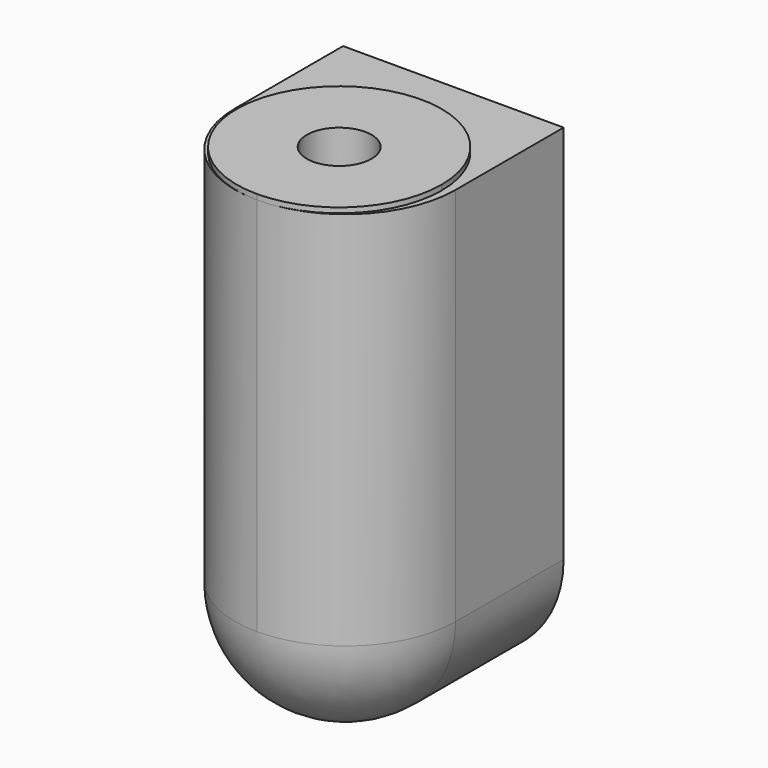
from build123d import *

# Parameters (mm, degrees)
F1_DEPTH = 18.9
F2_R     = 8.49999
F4_DEPTH = 0.4
F5_R     = 2.5
F6_DEPTH = 10
F7_R     = 2.5
F8_DEPTH = 25


# Not quite as in the source:
# - a fillet or chamfer is up to 0.001 mm smaller than in the source, because OpenCascade refuses the exact size


with BuildPart() as f1:
    # F0 (on Front) → F1 (new body)
    with BuildSketch(Plane.XZ):
        with BuildLine():
            ThreePointArc((-8.5, 0), (0, 8.5), (8.5, 0))
            Line((8.5, 0), (8.5, 29.3))
            Line((8.5, 29.3), (-8.5, 29.3))
            Line((-8.5, 29.3), (-8.5, 0))
        make_face()
        with BuildLine():
            Line((-8.5, 0), (8.5, 0))
            ThreePointArc((8.5, 0), (0, 8.5), (-8.5, 0))
        make_face()
        with BuildLine():
            ThreePointArc((-8.5, 0), (0, -8.5), (8.5, 0))
            Line((8.5, 0), (-8.5, 0))
        make_face()
    extrude(amount=F1_DEPTH)

    # F2 (radius 8.5 in the source; OpenCascade refuses exactly that, so slightly less here)
    f2_edges = [f1.edges().sort_by_distance(p)[0] for p in [
        (8.5, -18.9, 14.65),
    ]]
    fillet(f2_edges, radius=F2_R)

    # F3 (on face) → F4 (join)
    with BuildSketch(Plane.XY.offset(29.3)):
        with BuildLine():
            ThreePointArc((0, -18.9), (5.5861435714, -16.5861435714), (7.9, -11))
            ThreePointArc((7.9, -11), (-5.5861435714, -5.4138564286), (0, -18.9))
        make_face()
    extrude(amount=F4_DEPTH)

    # F5 (on face) → F6 (cut)
    with BuildSketch(Plane(origin=(0, 0, 0), x_dir=(-1, 0, 0), z_dir=(0, 1, 0))):
        with Locations((0, 20.5)):
            Circle(F5_R)
        with Locations((0, 1.5)):
            Circle(F5_R)
    extrude(amount=-F6_DEPTH, mode=Mode.SUBTRACT)

    # F7 (on face) → F8 (cut)
    with BuildSketch(Plane.XY.offset(29.7)):
        with Locations((0, -11)):
            Circle(F7_R)
    extrude(amount=-F8_DEPTH, mode=Mode.SUBTRACT)


solid = f1.part
